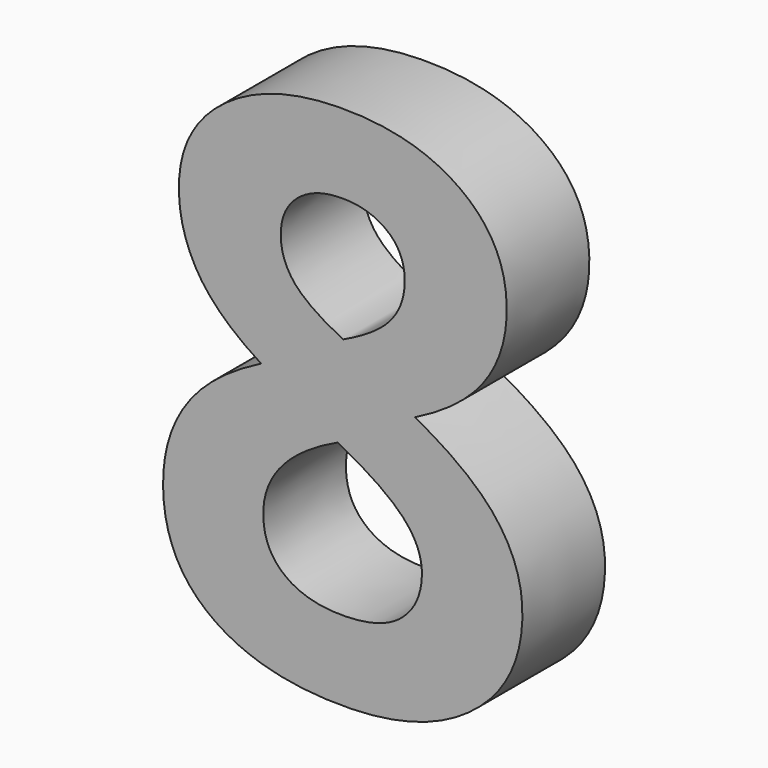
from build123d import *

# Parameters (mm, degrees)
F0_TEXT_SIZE = 35.2777777778
F1_DEPTH     = 5.08


# Not quite as in the source:
# - Text() gives the source's letters only with a copy of the font that has no kerning and outlines rounded to 1/6400 em; it was checked with that copy


with BuildPart() as f1:
    # F0 (on Front) → F1 (new body)
    with BuildSketch(Plane.XZ):
        with Locations((-69.7737952166, 9.6747119927)):
            Text('8', F0_TEXT_SIZE, font='Open Sans', font_style=FontStyle.BOLD, text_align=(TextAlign.LEFT, TextAlign.BOTTOM))
    extrude(amount=F1_DEPTH)


solid = f1.part
